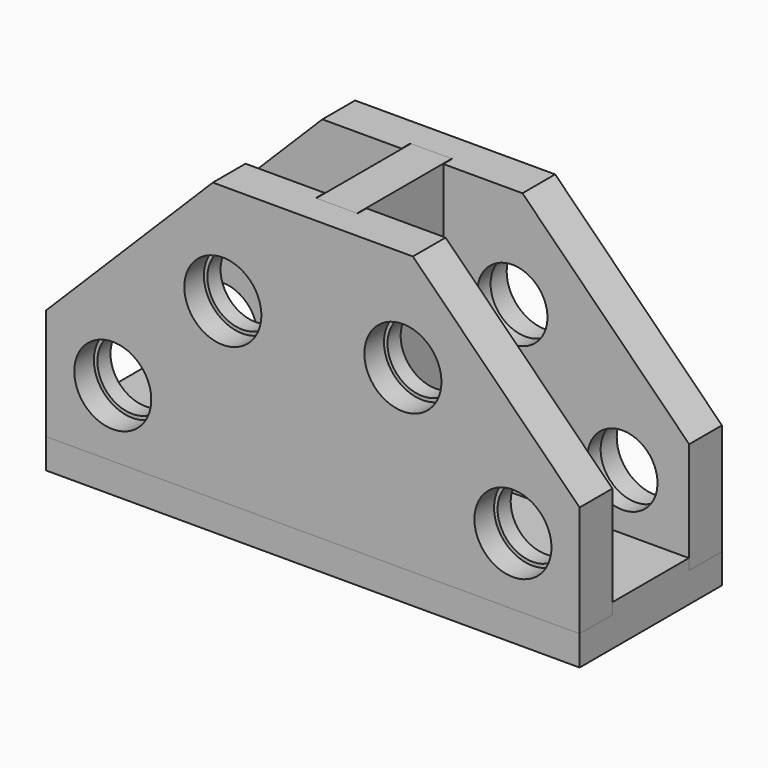
from build123d import *

# Parameters (mm, degrees)
F0_W      = 152.4
F0_H      = 50.8
F1_DEPTH  = 11.684
F3_DEPTH  = 11.684
F4_R      = 11
F5_DEPTH  = 7
F6_R      = 10
F7_DEPTH  = 4.684
F13_W     = 11.684
F13_H     = 33.782
F14_DEPTH = 79.375
F16_DEPTH = 3.175
F17_W     = 11.938
F17_H     = 33.782
F18_DEPTH = 79.375


with BuildPart() as f1:
    # F0 (on Top) → F1 (new body)
    with BuildSketch(Plane.XY):
        with Locations((0, 25.4)):
            Rectangle(F0_W, F0_H)
    extrude(amount=F1_DEPTH)

    # F15 (on face) → F16 (cut, through all)
    with BuildSketch(Plane.XY.offset(11.684)):
        Polygon((76.2, 50.8), (-76.2, 50.8), (-76.2, 38.989), (-5.969, 38.989), (-5.969, 11.811), (-76.2, 11.811), (-76.2, -0.127), (76.2, -0.127), (76.2, 11.811), (5.969, 11.811), (5.969, 38.989), (76.2, 38.989), align=None)
    extrude(amount=-F16_DEPTH, mode=Mode.SUBTRACT)


with BuildPart() as f3:
    # F2 (on face) → F3 (new body)
    with BuildSketch(Plane(origin=(0, 50.8, 0), x_dir=(-1, 0, 0), z_dir=(0, 1, 0))):
        Polygon((-76.2, 40.259), (-76.2, 8.509), (76.2, 8.509), (76.2, 40.259), (28.575, 87.884), (-28.575, 87.884), align=None)
    extrude(amount=-F3_DEPTH)

    # F4 (on face) → F5 (cut)
    with BuildSketch(Plane(origin=(0, 50.8, 0), x_dir=(-1, 0, 0), z_dir=(0, 1, 0))):
        with Locations((-57.15, 27.559)):
            Circle(F4_R)
        with Locations((-25.7191035763, 58.9898964237)):
            Circle(F4_R)
        with Locations((25.7191035763, 58.9898964237)):
            Circle(F4_R)
        with Locations((57.15, 27.559)):
            Circle(F4_R)
    extrude(amount=-F5_DEPTH, mode=Mode.SUBTRACT)

    # F6 (on face) → F7 (cut, through all)
    with BuildSketch(Plane(origin=(0, 43.8, 0), x_dir=(-1, 0, 0), z_dir=(0, 1, 0))):
        with Locations((-25.7191035763, 58.9898964237)):
            Circle(F6_R)
        with Locations((-57.15, 27.559)):
            Circle(F6_R)
        with Locations((25.7191035763, 58.9898964237)):
            Circle(F6_R)
        with Locations((57.15, 27.559)):
            Circle(F6_R)
    extrude(amount=-F7_DEPTH, mode=Mode.SUBTRACT)


with BuildPart() as f12_1:
    # F12: instance of F3
    add(f3.part.mirror(Plane(origin=(-76.2, 25.4, 11.684), x_dir=(0, 0, -1), z_dir=(0, 1, 0))))


with BuildPart() as f14:
    # F13 (on face) → F14 (new body, through all)
    with BuildSketch(Plane.XY.offset(87.884)):
        with Locations((0, 25.4)):
            Rectangle(F13_W, F13_H)
    extrude(amount=-F14_DEPTH)


with BuildPart() as f18_tool:
    # F17 (on face) → F18 (new body, through all)
    with BuildSketch(Plane.XY.offset(87.884)):
        with Locations((0, 25.4)):
            Rectangle(F17_W, F17_H)
    extrude(amount=-F18_DEPTH)


with BuildPart() as f3_1:
    add(f3.part)

    # F18: cut by f18_tool
    add(f18_tool.part, mode=Mode.SUBTRACT)


with BuildPart() as f12_1_1:
    add(f12_1.part)

    # F18: cut by f18_tool
    add(f18_tool.part, mode=Mode.SUBTRACT)


solid = Compound([f1.part, f14.part, f3_1.part, f12_1_1.part])
